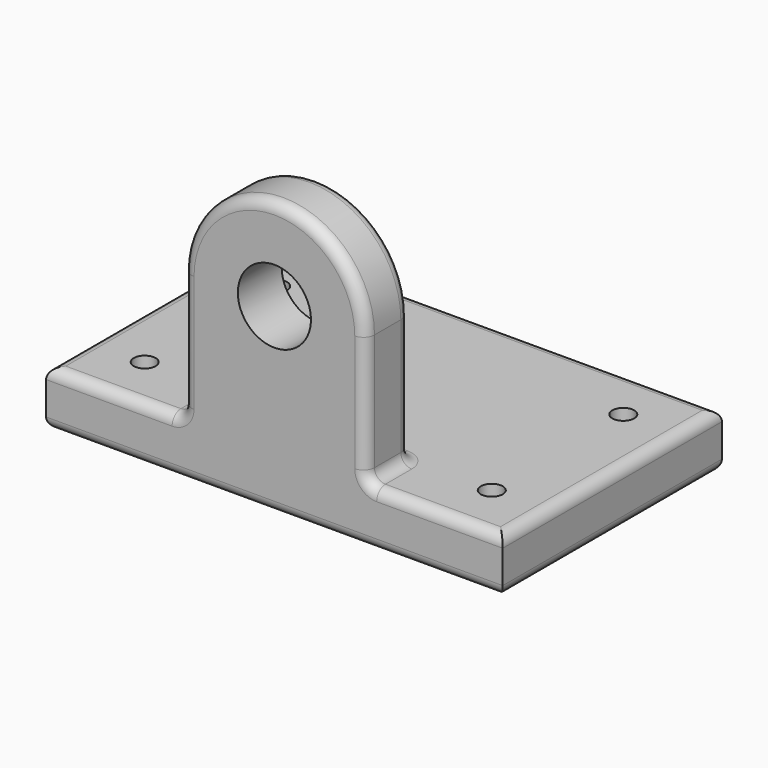
from build123d import *

# Parameters (mm, degrees)
F0_W     = 125
F0_H     = 75
F1_DEPTH = 15
F2_W     = 50
F2_H     = 15
F3_DEPTH = 15
F4_R     = 3
F5_DEPTH = 15.001
F6_R     = 3


with BuildPart() as f1:
    # F0 (on Top) → F1 (new body)
    with BuildSketch(Plane.XY):
        Rectangle(F0_W, F0_H)
    extrude(amount=F1_DEPTH)

    # F2 (on face) → F3 (join)
    with BuildSketch(Plane.XZ.offset(37.5)):
        with Locations((0, 7.5)):
            Rectangle(F2_W, F2_H)
        with BuildLine():
            Line((25, 15), (25, 50))
            ThreePointArc((25, 50), (0, 25), (-25, 50))
            Line((-25, 50), (-25, 15))
            Line((-25, 15), (25, 15))
        make_face()
        with BuildLine():
            ThreePointArc((-25, 50), (0, 25), (25, 50))
            Line((25, 50), (10, 50))
            ThreePointArc((10, 50), (0, 40), (-10, 50))
            Line((-10, 50), (-25, 50))
        make_face()
        with BuildLine():
            Line((10, 50), (25, 50))
            ThreePointArc((25, 50), (0, 75), (-25, 50))
            Line((-25, 50), (-10, 50))
            ThreePointArc((-10, 50), (0, 60), (10, 50))
        make_face()
    extrude(amount=-F3_DEPTH)

    # F4 (on face) → F5 (cut, through all)
    with BuildSketch(Plane.XY.offset(15)):
        with Locations((-47.5, 22.5)):
            Circle(F4_R)
        with Locations((-47.5, -22.5)):
            Circle(F4_R)
        with Locations((47.5, 22.5)):
            Circle(F4_R)
        with Locations((47.5, -22.5)):
            Circle(F4_R)
    extrude(amount=-F5_DEPTH, mode=Mode.SUBTRACT)

    # F6
    f6_edges = [f1.edges().sort_by_distance(p)[0] for p in [
        (-43.75, -37.5, 15),
        (-62.5, 0, 15),
        (0, 37.5, 15),
        (62.5, 0, 15),
        (43.75, -37.5, 15),
        (25, -30, 15),
        (-25, -30, 15),
        (-25, -22.5, 32.5),
        (0, -37.5, 0),
        (62.5, 0, 0),
        (0, 37.5, 0),
        (-62.5, 0, 0),
        (-25, -37.5, 32.5),
        (0, -37.5, 75),
        (25, -37.5, 32.5),
        (0, -22.5, 15),
        (0, -22.5, 75),
        (25, -22.5, 32.5),
    ]]
    fillet(f6_edges, radius=F6_R)


solid = f1.part
